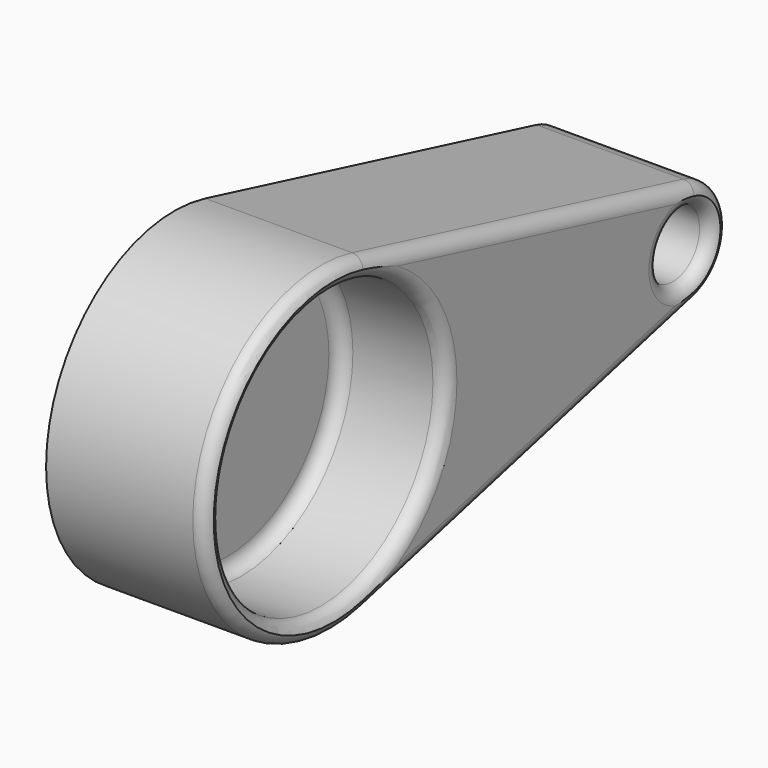
from build123d import *

# Parameters (mm, degrees)
F1_DEPTH    = 76.2
F2_R        = 66.675
F2_R_2      = 15.875
F3_DEPTH    = 50.8
F4_F1_R     = 6.35
F4_T2_DEPTH = 203.2
F4_T4_DEPTH = 203.2
F4_T7_ANGLE = 208.0724869359
F4_T9_ANGLE = 151.9275130641
F5_T        = -2.54


# Not quite as in the source:
# - a fillet or chamfer that OpenCascade refuses, or shapes differently, is made with other operations: its cross-section is extruded or revolved along the edge and cut away or added


with BuildPart() as f1:
    # F0 (on Right) → F1 (new body)
    with BuildSketch(Plane.YZ):
        with BuildLine():
            ThreePointArc((18.4812146278, -73.9248585111), (60.0612543768, -46.8944103565), (76.2, 0))
            ThreePointArc((76.2, 0), (60.0612543768, 46.8944103565), (18.4812146278, 73.9248585111))
            ThreePointArc((18.4812146278, 73.9248585111), (-76.2, 0), (18.4812146278, -73.9248585111))
        make_face()
        with BuildLine():
            ThreePointArc((18.4812146278, 73.9248585111), (60.0612543768, 46.8944103565), (76.2, 0))
            ThreePointArc((76.2, 0), (60.0612543768, -46.8944103565), (18.4812146278, -73.9248585111))
            Line((18.4812146278, -73.9248585111), (215.6141706573, -24.6416195037))
            ThreePointArc((215.6141706573, -24.6416195037), (184.0537657814, 0), (215.6141706573, 24.6416195037))
            Line((215.6141706573, 24.6416195037), (18.4812146278, 73.9248585111))
        make_face()
        with BuildLine():
            ThreePointArc((234.8537657814, 0), (229.474183907, 15.6314701188), (215.6141706573, 24.6416195037))
            ThreePointArc((215.6141706573, 24.6416195037), (184.0537657814, 0), (215.6141706573, -24.6416195037))
            ThreePointArc((215.6141706573, -24.6416195037), (229.474183907, -15.6314701188), (234.8537657814, 0))
        make_face()
    extrude(amount=F1_DEPTH)

    # F2 (on face) → F3 (cut)
    with BuildSketch(Plane.YZ.offset(76.2)):
        Circle(F2_R)
        with Locations((209.4537657814, 0)):
            Circle(F2_R_2)
    extrude(amount=-F3_DEPTH, mode=Mode.SUBTRACT)

    # F4: fillet of radius 6.35 on 8 edges, made by hand

    # F4_f1
    f4_f1_edges = [f1.edges().sort_by_distance(p)[0] for p in [
        (25.4, -66.675, 0),
        (25.4, 193.5787657814, 0),
    ]]
    fillet(f4_f1_edges, radius=F4_F1_R)

    # F4_s3 → F4_t2 (cut)
    with BuildSketch(Plane(origin=(0, 197.1329560295, -49.2832390074), x_dir=(1, 0, 0), z_dir=(0, -0.9701425001, 0.242535625))):
        with BuildLine():
            ThreePointArc((76.2, 69.85), (74.3401280605, 74.3401280605), (69.85, 76.2))
            Line((69.85, 76.2), (69.85, 76.327))
            Line((69.85, 76.327), (76.327, 76.327))
            Line((76.327, 76.327), (76.327, 69.85))
            Line((76.327, 69.85), (76.2, 69.85))
        make_face()
    extrude(amount=F4_T2_DEPTH, mode=Mode.SUBTRACT)

    # F4_s5 → F4_t4 (cut)
    with BuildSketch(Plane(origin=(0, 0, 0), x_dir=(1, 0, 0), z_dir=(0, 0.9701425001, 0.242535625))):
        with BuildLine():
            ThreePointArc((76.2, 69.85), (74.3401280605, 74.3401280605), (69.85, 76.2))
            Line((69.85, 76.2), (69.85, 76.327))
            Line((69.85, 76.327), (76.327, 76.327))
            Line((76.327, 76.327), (76.327, 69.85))
            Line((76.327, 69.85), (76.2, 69.85))
        make_face()
    extrude(amount=F4_T4_DEPTH, mode=Mode.SUBTRACT)

    # F4_s6 → F4_t7 (revolve, cut)
    with BuildSketch(Plane(origin=(0, 0, 0), x_dir=(1, 0, 0), z_dir=(0, 0.9701425001, -0.242535625))):
        with BuildLine():
            ThreePointArc((76.2, -69.85), (74.3401280605, -74.3401280605), (69.85, -76.2))
            Line((69.85, -76.2), (69.85, -76.327))
            Line((69.85, -76.327), (76.327, -76.327))
            Line((76.327, -76.327), (76.327, -69.85))
            Line((76.327, -69.85), (76.2, -69.85))
        make_face()
    revolve(axis=Axis((76.2, 0, 0), (1, 0, 0)), revolution_arc=F4_T7_ANGLE, mode=Mode.SUBTRACT)

    # F4_s8 → F4_t9 (revolve, cut)
    with BuildSketch(Plane(origin=(0, 197.1329560295, 49.2832390074), x_dir=(1, 0, 0), z_dir=(0, -0.9701425001, -0.242535625))):
        with BuildLine():
            ThreePointArc((76.2, -69.85), (74.3401280605, -74.3401280605), (69.85, -76.2))
            Line((69.85, -76.2), (69.85, -76.327))
            Line((69.85, -76.327), (76.327, -76.327))
            Line((76.327, -76.327), (76.327, -69.85))
            Line((76.327, -69.85), (76.2, -69.85))
        make_face()
    revolve(axis=Axis((76.2, 209.4537657814, 0), (1, 0, 0)), revolution_arc=F4_T9_ANGLE, mode=Mode.SUBTRACT)

    # F4_s10 → F4_t11 (revolve, cut)
    with BuildSketch(Plane.XY):
        with BuildLine():
            ThreePointArc((69.85, 225.3287657814), (74.3401280605, 227.1886377208), (76.2, 231.6787657814))
            Line((76.2, 231.6787657814), (76.327, 231.6787657814))
            Line((76.327, 231.6787657814), (76.327, 225.2017657814))
            Line((76.327, 225.2017657814), (69.85, 225.2017657814))
            Line((69.85, 225.2017657814), (69.85, 225.3287657814))
        make_face()
    revolve(axis=Axis((76.2, 209.4537657814, 0), (1, 0, 0)), mode=Mode.SUBTRACT)

    # F4_s12 → F4_t13 (revolve, cut)
    with BuildSketch(Plane.XY):
        with BuildLine():
            ThreePointArc((76.2, 73.025), (74.3401280605, 68.5348719395), (69.85, 66.675))
            Line((69.85, 66.675), (69.85, 66.548))
            Line((69.85, 66.548), (76.327, 66.548))
            Line((76.327, 66.548), (76.327, 73.025))
            Line((76.327, 73.025), (76.2, 73.025))
        make_face()
    revolve(axis=Axis((76.2, 0, 0), (1, 0, 0)), mode=Mode.SUBTRACT)

    # F5
    f5_openings = [f1.faces().sort_by_distance(p)[0] for p in [
        (0, 57.51924, 0),
    ]]
    offset(amount=F5_T, openings=f5_openings)


solid = f1.part
